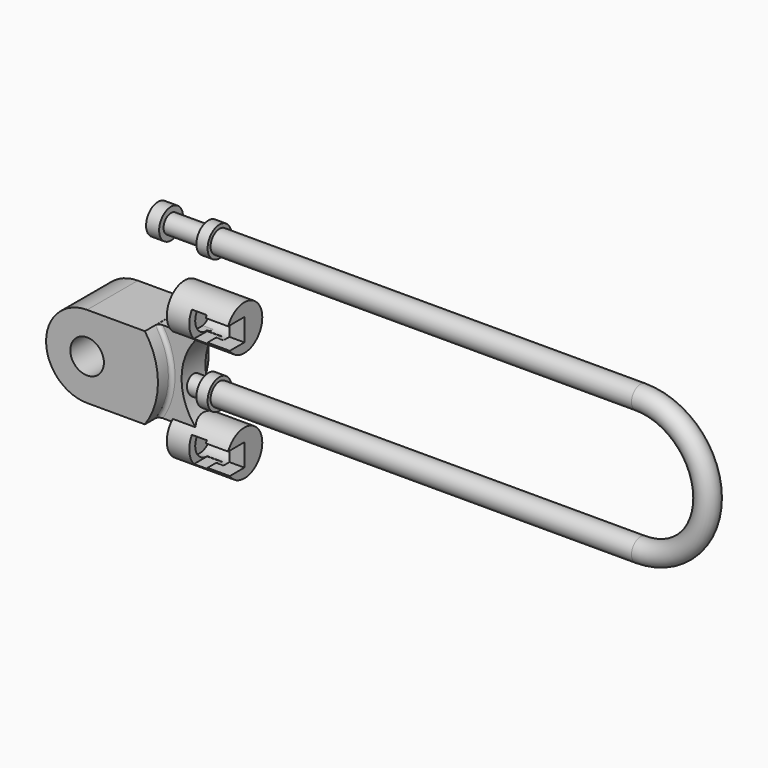
from build123d import *

# Parameters (mm, degrees)
F1_DEPTH      = 13.49375
F5_R          = 4.7625
F10_DEPTH     = 6.35
F11_T4_ANGLE  = 80.9473343059
F11_S5_R      = 30.5333867313
F11_T6_DEPTH  = 25
F11_T12_ANGLE = 80.9473343059
F11_S13_R     = 30.5333867313
F11_T14_DEPTH = 25
F13_R         = 9.525
F14_DEPTH     = 25.4
F17_R         = 6.35
F18_DEPTH     = 6.35
F20_DEPTH     = 25.4


# Not quite as in the source:
# - a fillet or chamfer that OpenCascade refuses, or shapes differently, is made with other operations: its cross-section is extruded or revolved along the edge and cut away or added


with BuildPart() as f1:
    # F0 (on Front) → F1 (new body, symmetric)
    with BuildSketch(Plane.XZ):
        with BuildLine():
            Line((24.5934442484, 17.4625), (0, 17.4625))
            ThreePointArc((0, 17.4625), (-17.4625, 0), (0, -17.4625))
            Line((0, -17.4625), (24.5934442484, -17.4625))
            ThreePointArc((24.5934442484, -17.4625), (30.1625, 0), (24.5934442484, 17.4625))
        make_face()
        with BuildLine():
            ThreePointArc((0, 7.14375), (5.0513940681, 5.0513940681), (7.14375, 0))
            ThreePointArc((7.14375, 0), (-5.0513940681, -5.0513940681), (0, 7.14375))
        make_face(mode=Mode.SUBTRACT)
    extrude(amount=F1_DEPTH, both=True)

    # F2 (on Front) → F10 (join, symmetric)
    with BuildSketch(Plane.XZ):
        with BuildLine():
            ThreePointArc((41.4273701276, -17.4469407648), (34.4871712628, 0), (41.4273701276, 17.4469407648))
            Line((41.4273701276, 17.4469407648), (24.6169958264, 17.4469407648))
            ThreePointArc((24.6169958264, 17.4469407648), (30.0926100463, 0), (24.6169958264, -17.4469407648))
            Line((24.6169958264, -17.4469407648), (41.4273701276, -17.4469407648))
        make_face()
    extrude(amount=F10_DEPTH, both=True)

    # F11: fillet of radius 1.5875 on 2 edges, made by hand


with BuildPart() as f4:
    # F3 (on Front) → F4 (revolve)
    with BuildSketch(Plane.XZ):
        Polygon((19.3847306073, 58.7863922119), (19.3847306073, 52.4363927543), (45.5784806073, 52.4363927543), (45.5784806073, 56.4051427543), (45.5784806073, 58.7863922119), (40.8159806073, 58.7863922119), (40.8159806073, 56.4051427543), (24.9409806073, 56.4051427543), (24.9409806073, 58.7863922119), align=None)
    revolve(axis=Axis((32.4938297272, 0, 52.4363927543), (1, 0, 0)))


with BuildPart() as f7:
    # F7: sweep along a path in F6
    with BuildLine(Plane.XZ) as f7_path:
        Line((45.5784806073, 52.4363927543), (224.7459987064, 52.4363927543))
        ThreePointArc((224.7459987064, 52.4363927543), (253.3209987064, 23.8613927543), (224.7459987064, -4.7136072457))
        Line((224.7459987064, -4.7136072457), (45.5784806073, -4.7136072457))
    # F5 (on face) → F7 (sweep)
    with BuildSketch(Plane.YZ.offset(45.5784806073)):
        with Locations((0, 52.4363927543)):
            Circle(F5_R)
    sweep(path=f7_path.line)


with BuildPart() as f8_1:
    # F8: copy of F4
    add(f4.part.moved(Location((0, 0, -57.15))))


with BuildPart() as f11_tool2:
    # F11_s3 → F11_t4 (revolve)
    with BuildSketch(Plane(origin=(0, 0, 0), x_dir=(0, 1, 0), z_dir=(-0.6490985011, 0, -0.7607043683))):
        with BuildLine():
            ThreePointArc((-7.9375, 30.1625), (-6.8149679849, 30.6274679849), (-6.35, 31.75))
            Line((-6.35, 31.75), (-6.35, 30.1625))
            Line((-6.35, 30.1625), (-7.9375, 30.1625))
        make_face()
    revolve(axis=Axis((0, -6.35, 0), (0, -1, 0)), revolution_arc=F11_T4_ANGLE)

    # F11_s5 → F11_t6 (cut, symmetric)
    with BuildSketch(Plane.XZ.offset(7.7)):
        with Locations((-0.440776685, 0)):
            Circle(F11_S5_R)
    extrude(amount=F11_T6_DEPTH, both=True, mode=Mode.SUBTRACT)

    split(bisect_by=Plane.XY.offset(17.4469407648), keep=Keep.BOTTOM)

    split(bisect_by=Plane.XY.offset(-17.4469407648), keep=Keep.TOP)


with BuildPart() as f1_1:
    add(f1.part)

    # F11_t1: union F11_tool2
    add(f11_tool2.part)


with BuildPart() as f11_tool10:
    # F11_s11 → F11_t12 (revolve)
    with BuildSketch(Plane(origin=(0, 0, 0), x_dir=(0, 1, 0), z_dir=(-0.6490985011, 0, -0.7607043683))):
        with BuildLine():
            ThreePointArc((7.9375, 30.1625), (6.8149679849, 30.6274679849), (6.35, 31.75))
            Line((6.35, 31.75), (6.35, 30.1625))
            Line((6.35, 30.1625), (7.9375, 30.1625))
        make_face()
    revolve(axis=Axis((0, 6.35, 0), (0, -1, 0)), revolution_arc=F11_T12_ANGLE)

    # F11_s13 → F11_t14 (cut, symmetric)
    with BuildSketch(Plane.XZ.offset(-7.7)):
        with Locations((-0.440776685, 0)):
            Circle(F11_S13_R)
    extrude(amount=F11_T14_DEPTH, both=True, mode=Mode.SUBTRACT)

    split(bisect_by=Plane.XY.offset(17.4469407648), keep=Keep.BOTTOM)

    split(bisect_by=Plane.XY.offset(-17.4469407648), keep=Keep.TOP)


with BuildPart() as f1_2:
    add(f1_1.part)

    # F11_t9: union F11_tool10
    add(f11_tool10.part)


with BuildPart() as f14:
    # F13 (on plane+point) → F14 (new body)
    with BuildSketch(Plane.YZ.offset(56.1482459307)):
        with Locations((0, 28.575)):
            Circle(F13_R)
    extrude(amount=-F14_DEPTH)


with BuildPart() as f14_1:
    # F15: moved
    add(f14.part.moved(Location((0, 0, -5.02753))))

    # F17 (on offset) → F18 (cut, symmetric)
    with BuildSketch(Plane.YZ.offset(43.4482459307)):
        with Locations((0, 23.54747)):
            Circle(F17_R)
    extrude(amount=F18_DEPTH, both=True, mode=Mode.SUBTRACT)


with BuildPart() as f20_tool:
    # F19 (on Front) → F20 (new body)
    with BuildSketch(Plane.XZ):
        Polygon((46.6506819159, 28.5149818759), (40.3006819159, 28.5149818759), (40.3006819159, 17.0944531906), (46.6506819159, 17.0944531906), (46.6506819159, 18.0422175333), (56.8106819159, 18.0422175333), (56.8106819159, 27.5672175333), (46.6506819159, 27.5672175333), align=None)
    extrude(amount=F20_DEPTH)


with BuildPart() as f1_3:
    add(f1_2.part)

    # F20: cut by f20_tool
    add(f20_tool.part, mode=Mode.SUBTRACT)


with BuildPart() as f14_2:
    add(f14_1.part)

    # F20: cut by f20_tool
    add(f20_tool.part, mode=Mode.SUBTRACT)


with BuildPart() as f21_1:
    # F21: copy of F14
    add(f14_2.part.moved(Location((0, 0, -46.92842))))


solid = Compound([f4.part, f7.part, f8_1.part, f1_3.part, f14_2.part, f21_1.part])
